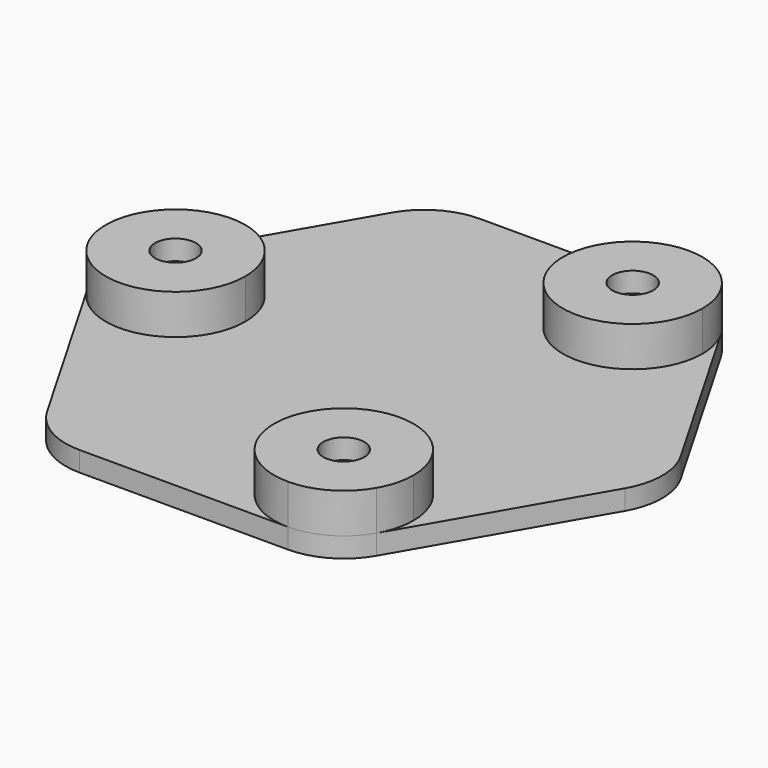
from build123d import *

# Parameters (mm, degrees)
F0_R     = 1.63322
F1_DEPTH = 1.5875
F2_R     = 5.55625
F3_R     = 1.63322
F4_DEPTH = 3.175
F6_R     = 3.175
F7_DEPTH = 3.175


# Not quite as in the source:
# - after a boolean that leaves OpenCascade's solid faulty, fix() repairs it
# - a pattern or mirror of a feature is missing from the dataset's text; its kind, count and spacing are read off the source's solid


with BuildPart() as f1:
    # F0 (on Top) → F1 (new body)
    with BuildSketch(Plane.XY):
        Polygon((11.5116069332, 19.938688085), (-11.5116069332, 19.938688085), (-23.0232138664, 0), (-11.5116069332, -19.938688085), (11.5116069332, -19.938688085), (23.0232138664, 0), align=None)
        with Locations((8.3037045, -14.382438085)):
            Circle(F0_R, mode=Mode.SUBTRACT)
        with Locations((-16.607409, 0)):
            Circle(F0_R, mode=Mode.SUBTRACT)
        with Locations((8.3037045, 14.382438085)):
            Circle(F0_R, mode=Mode.SUBTRACT)
    extrude(amount=F1_DEPTH)

    # F2
    f2_edges = [f1.edges().sort_by_distance(p)[0] for p in [
        (-23.023214, 0, 0.79375),
        (-11.511607, -19.938688, 0.79375),
        (11.511607, -19.938688, 0.79375),
        (23.023214, 0, 0.79375),
        (11.511607, 19.938688, 0.79375),
        (-11.511607, 19.938688, 0.79375),
    ]]
    fillet(f2_edges, radius=F2_R)

    # F3 (on face) → F4 (join)
    with BuildSketch(Plane.XY.offset(1.5875)):
        with BuildLine():
            ThreePointArc((13.1155581498, -17.160563085), (13.6706298723, -15.8205014044), (13.8599545, -14.382438085))
            ThreePointArc((13.8599545, -14.382438085), (4.374842447, -10.4535760321), (8.3037045, -19.938688085))
            ThreePointArc((8.3037045, -19.938688085), (11.0818295, -19.1942917348), (13.1155581498, -17.160563085))
        make_face()
        with Locations((8.3037045, -14.382438085)):
            Circle(F3_R, mode=Mode.SUBTRACT)
        with BuildLine():
            ThreePointArc((-21.4192626498, 2.778125), (-22.163659, 0), (-21.4192626498, -2.778125))
            ThreePointArc((-21.4192626498, -2.778125), (-15.1693456806, -5.3669253723), (-11.051159, 0))
            ThreePointArc((-11.051159, 0), (-15.1693456806, 5.3669253723), (-21.4192626498, 2.778125))
        make_face()
        with Locations((-16.607409, 0)):
            Circle(F3_R, mode=Mode.SUBTRACT)
    f4 = extrude(amount=F4_DEPTH)

    # F4_copies: F4 across plane
    add(f4.mirror(Plane.ZX))

    add(f1.part.fix(), mode=Mode.REPLACE)

    # F6 (on face) → F7 (cut, through all)
    with BuildSketch(Plane(origin=(0, 0, 0), x_dir=(1, 0, 0), z_dir=(0, 0, -1))):
        with Locations((8.3037045, 14.382438085)):
            Circle(F6_R)
        with Locations((8.3037045, -14.382438085)):
            Circle(F6_R)
        with Locations((-16.607409, 0)):
            Circle(F6_R)
    extrude(amount=-F7_DEPTH, mode=Mode.SUBTRACT)


solid = f1.part
